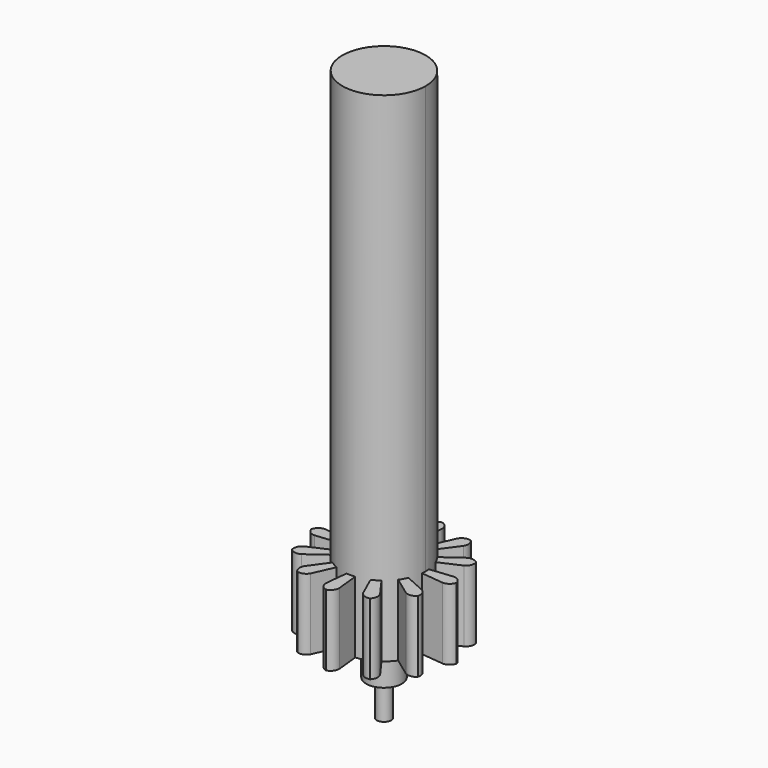
from build123d import *

# Parameters (mm, degrees)
F1_DEPTH        = 1
F1_COPIES_COUNT = 12
F3_DEPTH        = 7
F5_R            = 0.25
F6_DEPTH        = 0.5
F7_R            = 0.1
F8_DEPTH        = 0.5


# Not quite as in the source:
# - a feature of the source that left no trace in its solid (it failed there, or was rolled back) is left out
# - a pattern or mirror of a feature is missing from the dataset's text; its kind, count and spacing are read off the source's solid


with BuildPart() as f1:
    # F0 (on Top) → F1 (new body)
    with BuildSketch(Plane.XY):
        with BuildLine():
            ThreePointArc((0, 1.02075), (-0.0679119016, 0.9767079981), (-0.09375, 0.9))
            Line((-0.09375, 0.9), (-0.0606095593, 0.5818517692))
            ThreePointArc((-0.0606095593, 0.5818517692), (0, 0.585), (0.0606095593, 0.5818517692))
            Line((0.0606095593, 0.5818517692), (0.09375, 0.9))
            ThreePointArc((0.09375, 0.9), (0.0679119016, 0.9767079981), (0, 1.02075))
        make_face()
    extrude(amount=F1_DEPTH)


with BuildPart() as f1_copies_1:
    # F1_copies: instance of F1
    add(f1.part.rotate(Axis((0, 0, 0), (0, 0, 1)), 1 * 360 / F1_COPIES_COUNT))


with BuildPart() as f1_copies_2:
    # F1_copies: instance of F1
    add(f1.part.rotate(Axis((0, 0, 0), (0, 0, 1)), 2 * 360 / F1_COPIES_COUNT))


with BuildPart() as f1_copies_3:
    # F1_copies: instance of F1
    add(f1.part.rotate(Axis((0, 0, 0), (0, 0, 1)), 3 * 360 / F1_COPIES_COUNT))


with BuildPart() as f1_copies_4:
    # F1_copies: instance of F1
    add(f1.part.rotate(Axis((0, 0, 0), (0, 0, 1)), 4 * 360 / F1_COPIES_COUNT))


with BuildPart() as f1_copies_5:
    # F1_copies: instance of F1
    add(f1.part.rotate(Axis((0, 0, 0), (0, 0, 1)), 5 * 360 / F1_COPIES_COUNT))


with BuildPart() as f1_copies_6:
    # F1_copies: instance of F1
    add(f1.part.rotate(Axis((0, 0, 0), (0, 0, 1)), 6 * 360 / F1_COPIES_COUNT))


with BuildPart() as f1_copies_7:
    # F1_copies: instance of F1
    add(f1.part.rotate(Axis((0, 0, 0), (0, 0, 1)), 7 * 360 / F1_COPIES_COUNT))


with BuildPart() as f1_copies_8:
    # F1_copies: instance of F1
    add(f1.part.rotate(Axis((0, 0, 0), (0, 0, 1)), 8 * 360 / F1_COPIES_COUNT))


with BuildPart() as f1_copies_9:
    # F1_copies: instance of F1
    add(f1.part.rotate(Axis((0, 0, 0), (0, 0, 1)), 9 * 360 / F1_COPIES_COUNT))


with BuildPart() as f1_copies_10:
    # F1_copies: instance of F1
    add(f1.part.rotate(Axis((0, 0, 0), (0, 0, 1)), 10 * 360 / F1_COPIES_COUNT))


with BuildPart() as f1_copies_11:
    # F1_copies: instance of F1
    add(f1.part.rotate(Axis((0, 0, 0), (0, 0, 1)), 11 * 360 / F1_COPIES_COUNT))


with BuildPart() as f1_1:
    add(f1.part)

    add(f1_copies_1.part)  # F3 merges F1_copies_1

    add(f1_copies_2.part)  # F3 merges F1_copies_2

    add(f1_copies_3.part)  # F3 merges F1_copies_3

    add(f1_copies_4.part)  # F3 merges F1_copies_4

    add(f1_copies_5.part)  # F3 merges F1_copies_5

    add(f1_copies_6.part)  # F3 merges F1_copies_6

    add(f1_copies_7.part)  # F3 merges F1_copies_7

    add(f1_copies_8.part)  # F3 merges F1_copies_8

    add(f1_copies_9.part)  # F3 merges F1_copies_9

    add(f1_copies_10.part)  # F3 merges F1_copies_10

    add(f1_copies_11.part)  # F3 merges F1_copies_11
    # F0 (on Top) → F3 (join)
    with BuildSketch(Plane.XY):
        with BuildLine():
            ThreePointArc((0.0606095593, 0.5818517692), (0, 0.585), (-0.0606095593, 0.5818517692))
            ThreePointArc((-0.0606095593, 0.5818517692), (-0.3916429546, -0.4345581619), (0.585, 0))
            ThreePointArc((0.585, 0), (0.4345581619, 0.3916429546), (0.0606095593, 0.5818517692))
        make_face()
    extrude(amount=F3_DEPTH)

    # F4: union 

    # F5 (on face) → F6 (join)
    with BuildSketch(Plane(origin=(0, 0, 0), x_dir=(1, 0, 0), z_dir=(0, 0, -1))):
        Circle(F5_R)
    extrude(amount=F6_DEPTH)

    # F7 (on face) → F8 (join)
    with BuildSketch(Plane(origin=(0, 0, -0.5), x_dir=(1, 0, 0), z_dir=(0, 0, -1))):
        Circle(F7_R)
    extrude(amount=F8_DEPTH)


solid = f1_1.part
